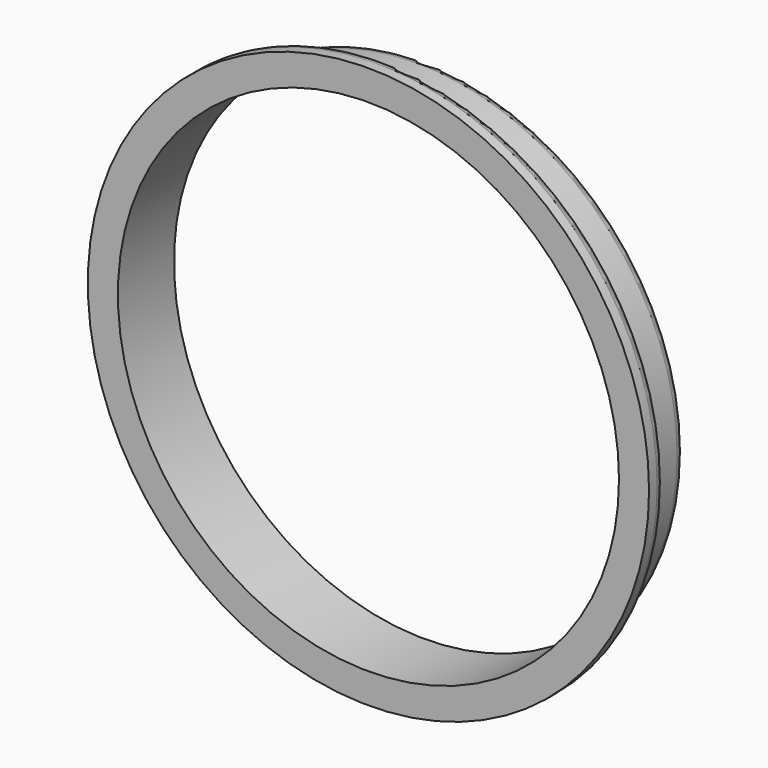
from build123d import *

# Parameters (mm, degrees)
F2_R = 0.99999
F3_R = 0.99999


# Not quite as in the source:
# - a fillet or chamfer is up to 0.001 mm smaller than in the source, because OpenCascade refuses the exact size


with BuildPart() as f1:
    # F0 (on Top) → F1 (revolve)
    with BuildSketch(Plane.XY):
        Polygon((25, 7), (25, 0), (28, 0), (28, 2), (26, 2), (26, 7), align=None)
    revolve(axis=Axis((0, 6.8999978745, 0), (0, 1, 0)))

    # F2 (radius 1 in the source; OpenCascade refuses exactly that, so slightly less here)
    f2_edges = [f1.edges().sort_by_distance(p)[0] for p in [
        (-26, 2, 0),
        (-28, 2, 0),
    ]]
    fillet(f2_edges, radius=F2_R)

    # F3 (radius 1 in the source; OpenCascade refuses exactly that, so slightly less here)
    f3_edges = [f1.edges().sort_by_distance(p)[0] for p in [
        (-26, 7, 0),
    ]]
    fillet(f3_edges, radius=F3_R)


solid = f1.part
